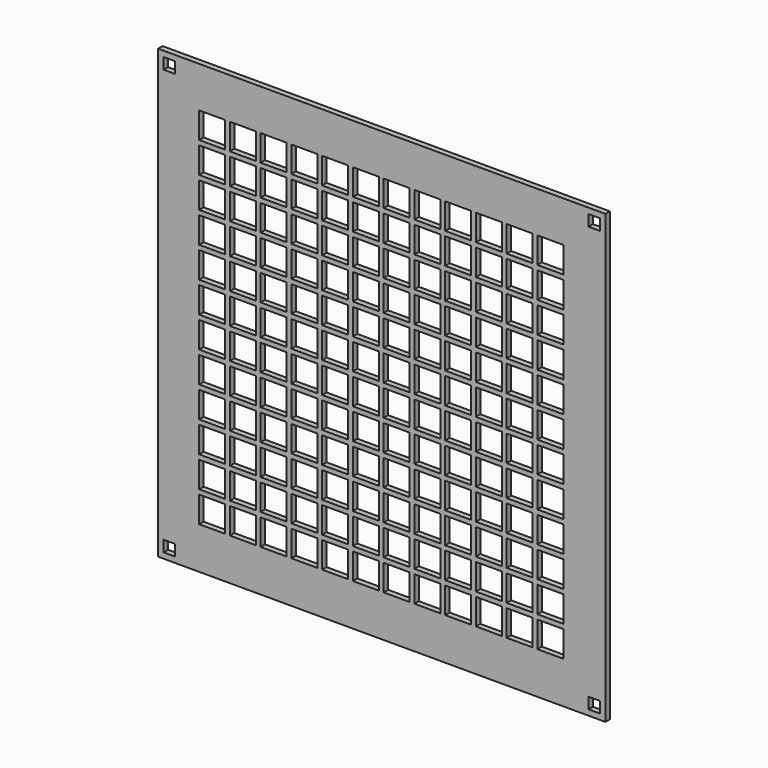
from build123d import *

# Parameters (mm, degrees)
F0_W     = 240
F0_H     = 240
F0_W_2   = 14
F0_H_2   = 14
F1_DEPTH = 3
F2_W     = 6
F2_H     = 6
F3_DEPTH = 3.001


with BuildPart() as f1:
    # F0 (on Front) → F1 (new body)
    with BuildSketch(Plane.XZ):
        with Locations((-12.5499347448, 36.2417517798)):
            Rectangle(F0_W, F0_H)
        with Locations((-103.5499347448, -54.2582482202)):
            Rectangle(F0_W_2, F0_H_2, mode=Mode.SUBTRACT)
        with Locations((-87.0499347448, -54.2582482202)):
            Rectangle(F0_W_2, F0_H_2, mode=Mode.SUBTRACT)
        with Locations((-103.5499347448, -37.7582482202)):
            Rectangle(F0_W_2, F0_H_2, mode=Mode.SUBTRACT)
        with Locations((-87.0499347448, -37.7582482202)):
            Rectangle(F0_W_2, F0_H_2, mode=Mode.SUBTRACT)
        with Locations((-70.5499347448, -54.2582482202)):
            Rectangle(F0_W_2, F0_H_2, mode=Mode.SUBTRACT)
        with Locations((-54.0499347448, -54.2582482202)):
            Rectangle(F0_W_2, F0_H_2, mode=Mode.SUBTRACT)
        with Locations((-37.5499347448, -54.2582482202)):
            Rectangle(F0_W_2, F0_H_2, mode=Mode.SUBTRACT)
        with Locations((-21.0499347448, -54.2582482202)):
            Rectangle(F0_W_2, F0_H_2, mode=Mode.SUBTRACT)
        with Locations((-70.5499347448, -37.7582482202)):
            Rectangle(F0_W_2, F0_H_2, mode=Mode.SUBTRACT)
        with Locations((-54.0499347448, -37.7582482202)):
            Rectangle(F0_W_2, F0_H_2, mode=Mode.SUBTRACT)
        with Locations((-37.5499347448, -37.7582482202)):
            Rectangle(F0_W_2, F0_H_2, mode=Mode.SUBTRACT)
        with Locations((-21.0499347448, -37.7582482202)):
            Rectangle(F0_W_2, F0_H_2, mode=Mode.SUBTRACT)
        with Locations((-103.5499347448, -21.2582482202)):
            Rectangle(F0_W_2, F0_H_2, mode=Mode.SUBTRACT)
        with Locations((-103.5499347448, -4.7582482202)):
            Rectangle(F0_W_2, F0_H_2, mode=Mode.SUBTRACT)
        with Locations((-87.0499347448, -21.2582482202)):
            Rectangle(F0_W_2, F0_H_2, mode=Mode.SUBTRACT)
        with Locations((-87.0499347448, -4.7582482202)):
            Rectangle(F0_W_2, F0_H_2, mode=Mode.SUBTRACT)
        with Locations((-103.5499347448, 11.7417517798)):
            Rectangle(F0_W_2, F0_H_2, mode=Mode.SUBTRACT)
        with Locations((-103.5499347448, 28.2417517798)):
            Rectangle(F0_W_2, F0_H_2, mode=Mode.SUBTRACT)
        with Locations((-87.0499347448, 11.7417517798)):
            Rectangle(F0_W_2, F0_H_2, mode=Mode.SUBTRACT)
        with Locations((-87.0499347448, 28.2417517798)):
            Rectangle(F0_W_2, F0_H_2, mode=Mode.SUBTRACT)
        with Locations((-70.5499347448, -21.2582482202)):
            Rectangle(F0_W_2, F0_H_2, mode=Mode.SUBTRACT)
        with Locations((-54.0499347448, -21.2582482202)):
            Rectangle(F0_W_2, F0_H_2, mode=Mode.SUBTRACT)
        with Locations((-70.5499347448, -4.7582482202)):
            Rectangle(F0_W_2, F0_H_2, mode=Mode.SUBTRACT)
        with Locations((-54.0499347448, -4.7582482202)):
            Rectangle(F0_W_2, F0_H_2, mode=Mode.SUBTRACT)
        with Locations((-37.5499347448, -21.2582482202)):
            Rectangle(F0_W_2, F0_H_2, mode=Mode.SUBTRACT)
        with Locations((-21.0499347448, -21.2582482202)):
            Rectangle(F0_W_2, F0_H_2, mode=Mode.SUBTRACT)
        with Locations((-37.5499347448, -4.7582482202)):
            Rectangle(F0_W_2, F0_H_2, mode=Mode.SUBTRACT)
        with Locations((-21.0499347448, -4.7582482202)):
            Rectangle(F0_W_2, F0_H_2, mode=Mode.SUBTRACT)
        with Locations((-70.5499347448, 11.7417517798)):
            Rectangle(F0_W_2, F0_H_2, mode=Mode.SUBTRACT)
        with Locations((-54.0499347448, 11.7417517798)):
            Rectangle(F0_W_2, F0_H_2, mode=Mode.SUBTRACT)
        with Locations((-70.5499347448, 28.2417517798)):
            Rectangle(F0_W_2, F0_H_2, mode=Mode.SUBTRACT)
        with Locations((-54.0499347448, 28.2417517798)):
            Rectangle(F0_W_2, F0_H_2, mode=Mode.SUBTRACT)
        with Locations((-37.5499347448, 11.7417517798)):
            Rectangle(F0_W_2, F0_H_2, mode=Mode.SUBTRACT)
        with Locations((-21.0499347448, 11.7417517798)):
            Rectangle(F0_W_2, F0_H_2, mode=Mode.SUBTRACT)
        with Locations((-37.5499347448, 28.2417517798)):
            Rectangle(F0_W_2, F0_H_2, mode=Mode.SUBTRACT)
        with Locations((-21.0499347448, 28.2417517798)):
            Rectangle(F0_W_2, F0_H_2, mode=Mode.SUBTRACT)
        with Locations((-4.5499347448, -54.2582482202)):
            Rectangle(F0_W_2, F0_H_2, mode=Mode.SUBTRACT)
        with Locations((11.9500652552, -54.2582482202)):
            Rectangle(F0_W_2, F0_H_2, mode=Mode.SUBTRACT)
        with Locations((28.4500652552, -54.2582482202)):
            Rectangle(F0_W_2, F0_H_2, mode=Mode.SUBTRACT)
        with Locations((44.9500652552, -54.2582482202)):
            Rectangle(F0_W_2, F0_H_2, mode=Mode.SUBTRACT)
        with Locations((-4.5499347448, -37.7582482202)):
            Rectangle(F0_W_2, F0_H_2, mode=Mode.SUBTRACT)
        with Locations((11.9500652552, -37.7582482202)):
            Rectangle(F0_W_2, F0_H_2, mode=Mode.SUBTRACT)
        with Locations((28.4500652552, -37.7582482202)):
            Rectangle(F0_W_2, F0_H_2, mode=Mode.SUBTRACT)
        with Locations((44.9500652552, -37.7582482202)):
            Rectangle(F0_W_2, F0_H_2, mode=Mode.SUBTRACT)
        with Locations((61.4500652552, -54.2582482202)):
            Rectangle(F0_W_2, F0_H_2, mode=Mode.SUBTRACT)
        with Locations((77.9500652552, -54.2582482202)):
            Rectangle(F0_W_2, F0_H_2, mode=Mode.SUBTRACT)
        with Locations((61.4500652552, -37.7582482202)):
            Rectangle(F0_W_2, F0_H_2, mode=Mode.SUBTRACT)
        with Locations((77.9500652552, -37.7582482202)):
            Rectangle(F0_W_2, F0_H_2, mode=Mode.SUBTRACT)
        with Locations((-4.5499347448, -21.2582482202)):
            Rectangle(F0_W_2, F0_H_2, mode=Mode.SUBTRACT)
        with Locations((11.9500652552, -21.2582482202)):
            Rectangle(F0_W_2, F0_H_2, mode=Mode.SUBTRACT)
        with Locations((-4.5499347448, -4.7582482202)):
            Rectangle(F0_W_2, F0_H_2, mode=Mode.SUBTRACT)
        with Locations((11.9500652552, -4.7582482202)):
            Rectangle(F0_W_2, F0_H_2, mode=Mode.SUBTRACT)
        with Locations((28.4500652552, -21.2582482202)):
            Rectangle(F0_W_2, F0_H_2, mode=Mode.SUBTRACT)
        with Locations((44.9500652552, -21.2582482202)):
            Rectangle(F0_W_2, F0_H_2, mode=Mode.SUBTRACT)
        with Locations((28.4500652552, -4.7582482202)):
            Rectangle(F0_W_2, F0_H_2, mode=Mode.SUBTRACT)
        with Locations((44.9500652552, -4.7582482202)):
            Rectangle(F0_W_2, F0_H_2, mode=Mode.SUBTRACT)
        with Locations((-4.5499347448, 11.7417517798)):
            Rectangle(F0_W_2, F0_H_2, mode=Mode.SUBTRACT)
        with Locations((11.9500652552, 11.7417517798)):
            Rectangle(F0_W_2, F0_H_2, mode=Mode.SUBTRACT)
        with Locations((-4.5499347448, 28.2417517798)):
            Rectangle(F0_W_2, F0_H_2, mode=Mode.SUBTRACT)
        with Locations((11.9500652552, 28.2417517798)):
            Rectangle(F0_W_2, F0_H_2, mode=Mode.SUBTRACT)
        with Locations((28.4500652552, 11.7417517798)):
            Rectangle(F0_W_2, F0_H_2, mode=Mode.SUBTRACT)
        with Locations((44.9500652552, 11.7417517798)):
            Rectangle(F0_W_2, F0_H_2, mode=Mode.SUBTRACT)
        with Locations((28.4500652552, 28.2417517798)):
            Rectangle(F0_W_2, F0_H_2, mode=Mode.SUBTRACT)
        with Locations((44.9500652552, 28.2417517798)):
            Rectangle(F0_W_2, F0_H_2, mode=Mode.SUBTRACT)
        with Locations((61.4500652552, -21.2582482202)):
            Rectangle(F0_W_2, F0_H_2, mode=Mode.SUBTRACT)
        with Locations((61.4500652552, -4.7582482202)):
            Rectangle(F0_W_2, F0_H_2, mode=Mode.SUBTRACT)
        with Locations((77.9500652552, -21.2582482202)):
            Rectangle(F0_W_2, F0_H_2, mode=Mode.SUBTRACT)
        with Locations((77.9500652552, -4.7582482202)):
            Rectangle(F0_W_2, F0_H_2, mode=Mode.SUBTRACT)
        with Locations((61.4500652552, 11.7417517798)):
            Rectangle(F0_W_2, F0_H_2, mode=Mode.SUBTRACT)
        with Locations((61.4500652552, 28.2417517798)):
            Rectangle(F0_W_2, F0_H_2, mode=Mode.SUBTRACT)
        with Locations((77.9500652552, 11.7417517798)):
            Rectangle(F0_W_2, F0_H_2, mode=Mode.SUBTRACT)
        with Locations((77.9500652552, 28.2417517798)):
            Rectangle(F0_W_2, F0_H_2, mode=Mode.SUBTRACT)
        with Locations((-103.5499347448, 44.7417517798)):
            Rectangle(F0_W_2, F0_H_2, mode=Mode.SUBTRACT)
        with Locations((-103.5499347448, 61.2417517798)):
            Rectangle(F0_W_2, F0_H_2, mode=Mode.SUBTRACT)
        with Locations((-87.0499347448, 44.7417517798)):
            Rectangle(F0_W_2, F0_H_2, mode=Mode.SUBTRACT)
        with Locations((-87.0499347448, 61.2417517798)):
            Rectangle(F0_W_2, F0_H_2, mode=Mode.SUBTRACT)
        with Locations((-103.5499347448, 77.7417517798)):
            Rectangle(F0_W_2, F0_H_2, mode=Mode.SUBTRACT)
        with Locations((-103.5499347448, 94.2417517798)):
            Rectangle(F0_W_2, F0_H_2, mode=Mode.SUBTRACT)
        with Locations((-87.0499347448, 77.7417517798)):
            Rectangle(F0_W_2, F0_H_2, mode=Mode.SUBTRACT)
        with Locations((-87.0499347448, 94.2417517798)):
            Rectangle(F0_W_2, F0_H_2, mode=Mode.SUBTRACT)
        with Locations((-70.5499347448, 44.7417517798)):
            Rectangle(F0_W_2, F0_H_2, mode=Mode.SUBTRACT)
        with Locations((-54.0499347448, 44.7417517798)):
            Rectangle(F0_W_2, F0_H_2, mode=Mode.SUBTRACT)
        with Locations((-70.5499347448, 61.2417517798)):
            Rectangle(F0_W_2, F0_H_2, mode=Mode.SUBTRACT)
        with Locations((-54.0499347448, 61.2417517798)):
            Rectangle(F0_W_2, F0_H_2, mode=Mode.SUBTRACT)
        with Locations((-37.5499347448, 44.7417517798)):
            Rectangle(F0_W_2, F0_H_2, mode=Mode.SUBTRACT)
        with Locations((-21.0499347448, 44.7417517798)):
            Rectangle(F0_W_2, F0_H_2, mode=Mode.SUBTRACT)
        with Locations((-37.5499347448, 61.2417517798)):
            Rectangle(F0_W_2, F0_H_2, mode=Mode.SUBTRACT)
        with Locations((-21.0499347448, 61.2417517798)):
            Rectangle(F0_W_2, F0_H_2, mode=Mode.SUBTRACT)
        with Locations((-70.5499347448, 77.7417517798)):
            Rectangle(F0_W_2, F0_H_2, mode=Mode.SUBTRACT)
        with Locations((-54.0499347448, 77.7417517798)):
            Rectangle(F0_W_2, F0_H_2, mode=Mode.SUBTRACT)
        with Locations((-70.5499347448, 94.2417517798)):
            Rectangle(F0_W_2, F0_H_2, mode=Mode.SUBTRACT)
        with Locations((-54.0499347448, 94.2417517798)):
            Rectangle(F0_W_2, F0_H_2, mode=Mode.SUBTRACT)
        with Locations((-37.5499347448, 77.7417517798)):
            Rectangle(F0_W_2, F0_H_2, mode=Mode.SUBTRACT)
        with Locations((-21.0499347448, 77.7417517798)):
            Rectangle(F0_W_2, F0_H_2, mode=Mode.SUBTRACT)
        with Locations((-37.5499347448, 94.2417517798)):
            Rectangle(F0_W_2, F0_H_2, mode=Mode.SUBTRACT)
        with Locations((-21.0499347448, 94.2417517798)):
            Rectangle(F0_W_2, F0_H_2, mode=Mode.SUBTRACT)
        with Locations((-103.5499347448, 110.7417517798)):
            Rectangle(F0_W_2, F0_H_2, mode=Mode.SUBTRACT)
        with Locations((-87.0499347448, 110.7417517798)):
            Rectangle(F0_W_2, F0_H_2, mode=Mode.SUBTRACT)
        with Locations((-103.5499347448, 127.2417517798)):
            Rectangle(F0_W_2, F0_H_2, mode=Mode.SUBTRACT)
        with Locations((-87.0499347448, 127.2417517798)):
            Rectangle(F0_W_2, F0_H_2, mode=Mode.SUBTRACT)
        with Locations((-70.5499347448, 110.7417517798)):
            Rectangle(F0_W_2, F0_H_2, mode=Mode.SUBTRACT)
        with Locations((-54.0499347448, 110.7417517798)):
            Rectangle(F0_W_2, F0_H_2, mode=Mode.SUBTRACT)
        with Locations((-37.5499347448, 110.7417517798)):
            Rectangle(F0_W_2, F0_H_2, mode=Mode.SUBTRACT)
        with Locations((-21.0499347448, 110.7417517798)):
            Rectangle(F0_W_2, F0_H_2, mode=Mode.SUBTRACT)
        with Locations((-70.5499347448, 127.2417517798)):
            Rectangle(F0_W_2, F0_H_2, mode=Mode.SUBTRACT)
        with Locations((-54.0499347448, 127.2417517798)):
            Rectangle(F0_W_2, F0_H_2, mode=Mode.SUBTRACT)
        with Locations((-37.5499347448, 127.2417517798)):
            Rectangle(F0_W_2, F0_H_2, mode=Mode.SUBTRACT)
        with Locations((-21.0499347448, 127.2417517798)):
            Rectangle(F0_W_2, F0_H_2, mode=Mode.SUBTRACT)
        with Locations((-4.5499347448, 44.7417517798)):
            Rectangle(F0_W_2, F0_H_2, mode=Mode.SUBTRACT)
        with Locations((11.9500652552, 44.7417517798)):
            Rectangle(F0_W_2, F0_H_2, mode=Mode.SUBTRACT)
        with Locations((-4.5499347448, 61.2417517798)):
            Rectangle(F0_W_2, F0_H_2, mode=Mode.SUBTRACT)
        with Locations((11.9500652552, 61.2417517798)):
            Rectangle(F0_W_2, F0_H_2, mode=Mode.SUBTRACT)
        with Locations((28.4500652552, 44.7417517798)):
            Rectangle(F0_W_2, F0_H_2, mode=Mode.SUBTRACT)
        with Locations((44.9500652552, 44.7417517798)):
            Rectangle(F0_W_2, F0_H_2, mode=Mode.SUBTRACT)
        with Locations((28.4500652552, 61.2417517798)):
            Rectangle(F0_W_2, F0_H_2, mode=Mode.SUBTRACT)
        with Locations((44.9500652552, 61.2417517798)):
            Rectangle(F0_W_2, F0_H_2, mode=Mode.SUBTRACT)
        with Locations((-4.5499347448, 77.7417517798)):
            Rectangle(F0_W_2, F0_H_2, mode=Mode.SUBTRACT)
        with Locations((11.9500652552, 77.7417517798)):
            Rectangle(F0_W_2, F0_H_2, mode=Mode.SUBTRACT)
        with Locations((-4.5499347448, 94.2417517798)):
            Rectangle(F0_W_2, F0_H_2, mode=Mode.SUBTRACT)
        with Locations((11.9500652552, 94.2417517798)):
            Rectangle(F0_W_2, F0_H_2, mode=Mode.SUBTRACT)
        with Locations((28.4500652552, 77.7417517798)):
            Rectangle(F0_W_2, F0_H_2, mode=Mode.SUBTRACT)
        with Locations((44.9500652552, 77.7417517798)):
            Rectangle(F0_W_2, F0_H_2, mode=Mode.SUBTRACT)
        with Locations((28.4500652552, 94.2417517798)):
            Rectangle(F0_W_2, F0_H_2, mode=Mode.SUBTRACT)
        with Locations((44.9500652552, 94.2417517798)):
            Rectangle(F0_W_2, F0_H_2, mode=Mode.SUBTRACT)
        with Locations((61.4500652552, 44.7417517798)):
            Rectangle(F0_W_2, F0_H_2, mode=Mode.SUBTRACT)
        with Locations((61.4500652552, 61.2417517798)):
            Rectangle(F0_W_2, F0_H_2, mode=Mode.SUBTRACT)
        with Locations((77.9500652552, 44.7417517798)):
            Rectangle(F0_W_2, F0_H_2, mode=Mode.SUBTRACT)
        with Locations((77.9500652552, 61.2417517798)):
            Rectangle(F0_W_2, F0_H_2, mode=Mode.SUBTRACT)
        with Locations((61.4500652552, 77.7417517798)):
            Rectangle(F0_W_2, F0_H_2, mode=Mode.SUBTRACT)
        with Locations((61.4500652552, 94.2417517798)):
            Rectangle(F0_W_2, F0_H_2, mode=Mode.SUBTRACT)
        with Locations((77.9500652552, 77.7417517798)):
            Rectangle(F0_W_2, F0_H_2, mode=Mode.SUBTRACT)
        with Locations((77.9500652552, 94.2417517798)):
            Rectangle(F0_W_2, F0_H_2, mode=Mode.SUBTRACT)
        with Locations((-4.5499347448, 110.7417517798)):
            Rectangle(F0_W_2, F0_H_2, mode=Mode.SUBTRACT)
        with Locations((11.9500652552, 110.7417517798)):
            Rectangle(F0_W_2, F0_H_2, mode=Mode.SUBTRACT)
        with Locations((28.4500652552, 110.7417517798)):
            Rectangle(F0_W_2, F0_H_2, mode=Mode.SUBTRACT)
        with Locations((44.9500652552, 110.7417517798)):
            Rectangle(F0_W_2, F0_H_2, mode=Mode.SUBTRACT)
        with Locations((-4.5499347448, 127.2417517798)):
            Rectangle(F0_W_2, F0_H_2, mode=Mode.SUBTRACT)
        with Locations((11.9500652552, 127.2417517798)):
            Rectangle(F0_W_2, F0_H_2, mode=Mode.SUBTRACT)
        with Locations((28.4500652552, 127.2417517798)):
            Rectangle(F0_W_2, F0_H_2, mode=Mode.SUBTRACT)
        with Locations((44.9500652552, 127.2417517798)):
            Rectangle(F0_W_2, F0_H_2, mode=Mode.SUBTRACT)
        with Locations((61.4500652552, 110.7417517798)):
            Rectangle(F0_W_2, F0_H_2, mode=Mode.SUBTRACT)
        with Locations((77.9500652552, 110.7417517798)):
            Rectangle(F0_W_2, F0_H_2, mode=Mode.SUBTRACT)
        with Locations((61.4500652552, 127.2417517798)):
            Rectangle(F0_W_2, F0_H_2, mode=Mode.SUBTRACT)
        with Locations((77.9500652552, 127.2417517798)):
            Rectangle(F0_W_2, F0_H_2, mode=Mode.SUBTRACT)
    extrude(amount=F1_DEPTH)

    # F2 (on face) → F3 (cut, through all)
    with BuildSketch(Plane.XZ.offset(3)):
        with Locations((-126.5499347448, 150.2417517798)):
            Rectangle(F2_W, F2_H)
        with Locations((101.4500652552, 150.2417517798)):
            Rectangle(F2_W, F2_H)
        with Locations((101.4500652552, -77.7582482202)):
            Rectangle(F2_W, F2_H)
        with Locations((-126.5499347448, -77.7582482202)):
            Rectangle(F2_W, F2_H)
    extrude(amount=-F3_DEPTH, mode=Mode.SUBTRACT)


solid = f1.part
